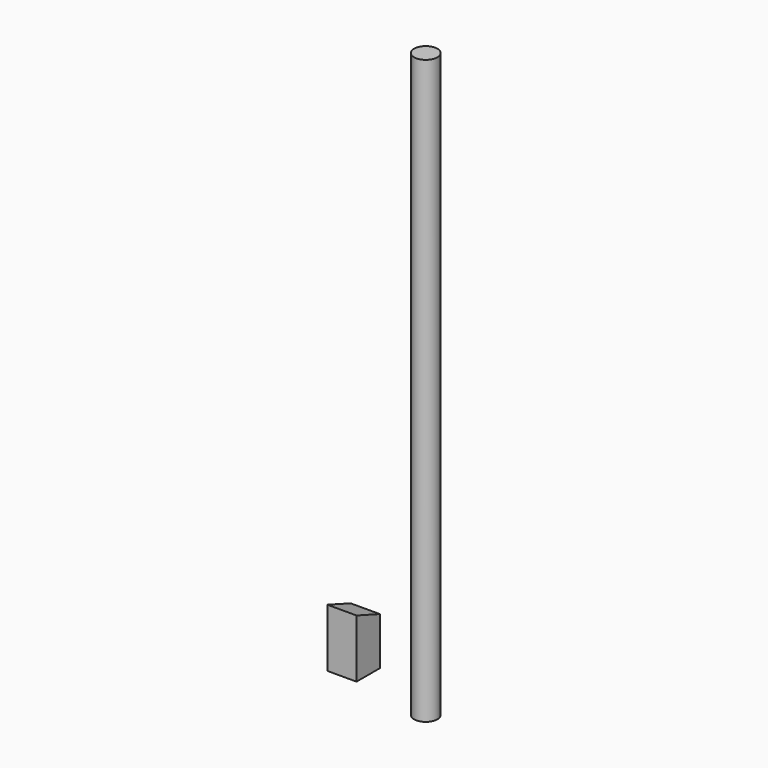
from build123d import *

# Parameters (mm, degrees)
F0_R     = 4
F1_DEPTH = 200
F2_W     = 10
F2_H     = 10
F3_DEPTH = 20
F4_SIZE2 = 3.639692
F4_SIZE  = 9.99999


# Not quite as in the source:
# - a fillet or chamfer is up to 0.001 mm smaller than in the source, because OpenCascade refuses the exact size


with BuildPart() as f1:
    # F0 (on Top) → F1 (new body)
    with BuildSketch(Plane.XY):
        Circle(F0_R)
    extrude(amount=F1_DEPTH)


with BuildPart() as f3:
    # F2 (on Top) → F3 (new body)
    with BuildSketch(Plane.XY):
        with Locations((-31.5685559809, 8.5248657316)):
            Rectangle(F2_W, F2_H)
    extrude(amount=F3_DEPTH)

    # F4 (size 10 and 3.6397023427 in the source; OpenCascade refuses exactly that, so slightly less here)
    f4_edges = [f3.edges().sort_by_distance(p)[0] for p in [
        (-31.568556, 13.524866, 20),
    ]]
    f4_side = f3.faces().sort_by_distance((-31.568556, 8.524866, 20))[0]
    chamfer(f4_edges, length=F4_SIZE, length2=F4_SIZE2, reference=f4_side)


solid = Compound([f1.part, f3.part])
